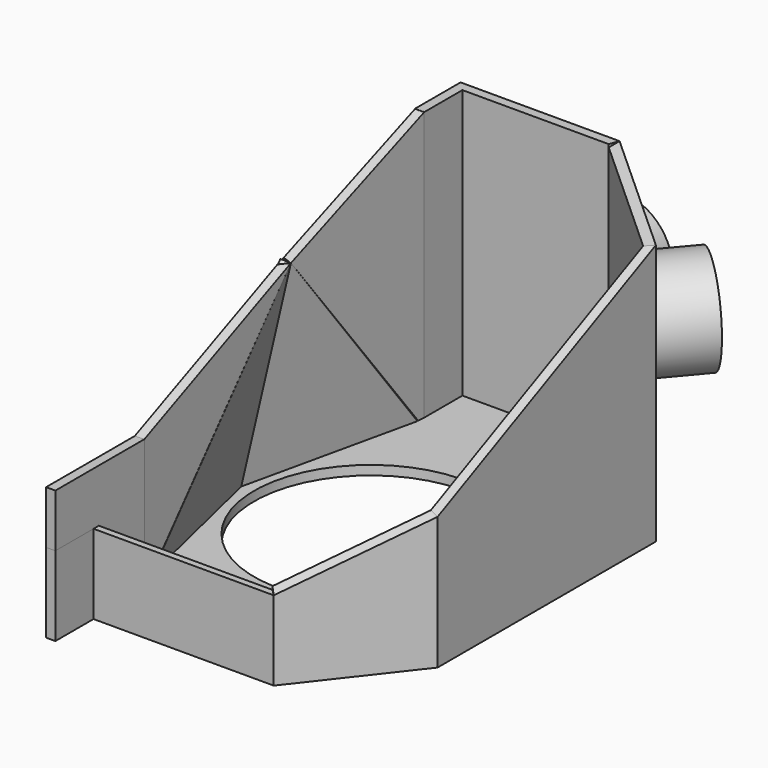
from build123d import *

# Parameters (mm, degrees)
F0_W      = 3.5
F0_H      = 18
F6_DEPTH  = 30
F7_REACH  = 201.50633824
F8_DEPTH  = 105
F10_REACH = 161.9332117682
F12_REACH = 102.7827771036
F15_DEPTH = 25
F16_DEPTH = 25
F0_R      = 5
F0_R_2    = 44
F17_DEPTH = 3.5
F21_DEPTH = 3.5
F0_H_2    = 21.5
F22_DEPTH = 50
F26_DEPTH = 3.5
F30_DEPTH = 3.5
F34_DEPTH = 3.5
F35_W     = 3.5
F35_H     = 20
F36_DEPTH = 20.5


with BuildPart() as f6:
    # F0 (on Top) → F6 (new body, through all)
    with BuildSketch(Plane.XY):
        Polygon((3.5, -177.5), (71.5, -177.5), (69.0107278246, -175), (3.5, -175), (0, -175), (0, -177.5), align=None)
        with Locations((1.75, -186.5)):
            Rectangle(F0_W, F0_H)
    extrude(amount=F6_DEPTH)



with BuildPart() as f7:
    f7_end = Plane(origin=(0, -44.3168900323, 94.2741115233), x_dir=(0, -0.9049939228, -0.4254244936), z_dir=(0, 0.4254244936, -0.9049939228))
    # F0 (on Top) → F7 (new body, up to a plane its end follows)
    with BuildSketch(Plane.XY):
        Polygon((102, -138.3286694261), (102, -35.3643643935), (98.5, -36.9928108308), (98.5, -137.1267531552), align=None)
    f7_long = extrude(amount=F7_REACH, mode=Mode.PRIVATE)
    add(split(f7_long, bisect_by=f7_end, keep=Keep.TOP, mode=Mode.PRIVATE))



with BuildPart() as f8:
    # F0 (on Top) → F8 (new body, through all)
    with BuildSketch(Plane.XY):
        Polygon((60, 0), (0, 0), (0, -21.5), (3.5, -21.5), (3.5, -3.5), (58.722724796, -3.5), align=None)
    extrude(amount=F8_DEPTH)


with BuildPart() as f7_1:
    add(f7.part)

    add(f8.part)  # F10 merges F8
    f10_end = Plane(origin=(60, 0, 105), x_dir=(0, 0.9614490001, 0.2749833091), z_dir=(-0.0820657574, -0.2740557675, 0.9582059527))
    # F0 (on Top) → F10 (join, up to a plane its end follows)
    with BuildSketch(Plane.XY):
        Polygon((102, -35.3643643935), (60, 0), (58.722724796, -3.5), (98.5, -36.9928108308), align=None)
    f10_long = extrude(amount=F10_REACH, mode=Mode.PRIVATE)
    add(split(f10_long, bisect_by=f10_end, keep=Keep.BOTTOM, mode=Mode.PRIVATE))


with BuildPart() as f6_1:
    add(f6.part)

    add(f7_1.part)  # F12 merges F7
    f12_end = Plane(origin=(98.5, -137.1267531552, 50.6455433886), x_dir=(0, 0.8931169065, 0.4498246228), z_dir=(-0.0102958733, -0.4498007803, 0.8930695679))
    # F0 (on Top) → F12 (join, up to a plane its end follows)
    with BuildSketch(Plane.XY):
        Polygon((71.5, -177.5), (102, -138.3286694261), (98.5, -137.1267531552), (69.0107278246, -175), align=None)
    f12_long = extrude(amount=F12_REACH, mode=Mode.PRIVATE)
    add(split(f12_long, bisect_by=f12_end, keep=Keep.BOTTOM, mode=Mode.PRIVATE))


with BuildPart() as f15:
    # F13 (on face) → F15 (new body)
    with BuildSketch(Plane(origin=(0, 0, 0), x_dir=(-1, 0, 0), z_dir=(0, 1, 0))):
        with BuildLine():
            ThreePointArc((-60, 52.5), (-41, 33.5), (-22, 52.5))
            ThreePointArc((-22, 52.5), (-41, 71.5), (-60, 52.5))
        make_face()
    extrude(amount=F15_DEPTH)


with BuildPart() as f16:
    # F14 (on face) → F16 (new body)
    with BuildSketch(Plane(origin=(24.8913101482, 29.5618214594, 0), x_dir=(-0.7649476001, 0.644092516, 0), z_dir=(0.644092516, 0.7649476001, 0))):
        with BuildLine():
            Line((-45.8968560046, 35.7509940048), (-45.8968560046, 68.0619828476))
            ThreePointArc((-45.8968560046, 68.0619828476), (-74.8968560046, 51.9064884262), (-45.8968560046, 35.7509940048))
        make_face()
        with BuildLine():
            ThreePointArc((-45.8968560046, 35.7509940048), (-39.2986633319, 42.6598674217), (-36.8968560046, 51.9064884262))
            ThreePointArc((-36.8968560046, 51.9064884262), (-39.2986633319, 61.1531094306), (-45.8968560046, 68.0619828476))
            Line((-45.8968560046, 68.0619828476), (-45.8968560046, 35.7509940048))
        make_face()
    extrude(amount=F16_DEPTH)


with BuildPart() as f17:
    # F0 (on Top) → F17 (new body)
    with BuildSketch(Plane.XY):
        Polygon((98.5, -36.9928108308), (58.722724796, -3.5), (3.5, -3.5), (3.5, -21.5), (3.5, -21.8849541017), (-11.5, -89.25), (3.5, -153.094366445), (3.5, -153.5), (3.5, -175), (69.0107278246, -175), (98.5, -137.1267531552), align=None)
        with Locations((37.5, -154.25)):
            Circle(F0_R, mode=Mode.SUBTRACT)
        with Locations((37.5, -89.25)):
            Circle(F0_R_2, mode=Mode.SUBTRACT)
        with Locations((37.5, -24.25)):
            Circle(F0_R, mode=Mode.SUBTRACT)
    extrude(amount=F17_DEPTH)


with BuildPart() as f21:
    # F20 (on 3pt) → F21 (new body)
    with BuildSketch(Plane(origin=(7.8663280231, -1.7515748527, -0.9582026436), x_dir=(-0.2142407567, -0.9764322069, 0.0260968089), z_dir=(-0.9692677662, 0.2158243389, 0.1180671507))):
        Polygon((80.1370792473, 76.9313541176), (20.619331384, 0.4232091326), (90.4000018708, -1.8246819942), align=None)
    extrude(amount=F21_DEPTH)


with BuildPart() as f22:
    # F0 (on Top) → F22 (new body)
    with BuildSketch(Plane.XY):
        with Locations((1.75, -164.25)):
            Rectangle(F0_W, F0_H_2)
    extrude(amount=F22_DEPTH)

    # F35 (on face) → F36 (join, through all)
    with BuildSketch(Plane.XZ.offset(175)):
        with Locations((1.75, 40)):
            Rectangle(F35_W, F35_H)
    extrude(amount=F36_DEPTH)


with BuildPart() as f26:
    # F25 (on 3pt) → F26 (new body)
    with BuildSketch(Plane(origin=(-30.3997140605, -7.2539765203, 5.5066874197), x_dir=(-0.2249220316, 0.9735245699, 0.0407429925), z_dir=(0.9579352039, 0.228582396, -0.1735230051))):
        Polygon((-149.8283543617, 0.623847139), (-85.0179586872, -2.493068384), (-74.7243836748, 76.2589672614), align=None)
    extrude(amount=-F26_DEPTH)


with BuildPart() as f30:
    # F29 (on 3pt) → F30 (new body)
    with BuildSketch(Plane(origin=(4.7692531664, -0.285339933, 0), x_dir=(-0.0597222669, -0.9982150324, 0), z_dir=(-0.9982150324, 0.0597222669, 0))):
        Polygon((79.8572025891, 77.5), (21.2525952617, 105.0000000001), (21.2525952617, 0), align=None)
    extrude(amount=F30_DEPTH)


with BuildPart() as f34:
    # F33 (on 3pt) → F34 (new body)
    with BuildSketch(Plane(origin=(-3.8009049774, -0.1809954751, 0), x_dir=(0.0475651494, -0.9988681377, 0), z_dir=(-0.9988681377, -0.0475651494, 0))):
        Polygon((153.4927371637, 50), (79.909451018, 77.5), (153.4927371637, 0), align=None)
    extrude(amount=F34_DEPTH)


solid = Compound([f6_1.part, f15.part, f16.part, f17.part, f21.part, f22.part, f26.part, f30.part, f34.part])
